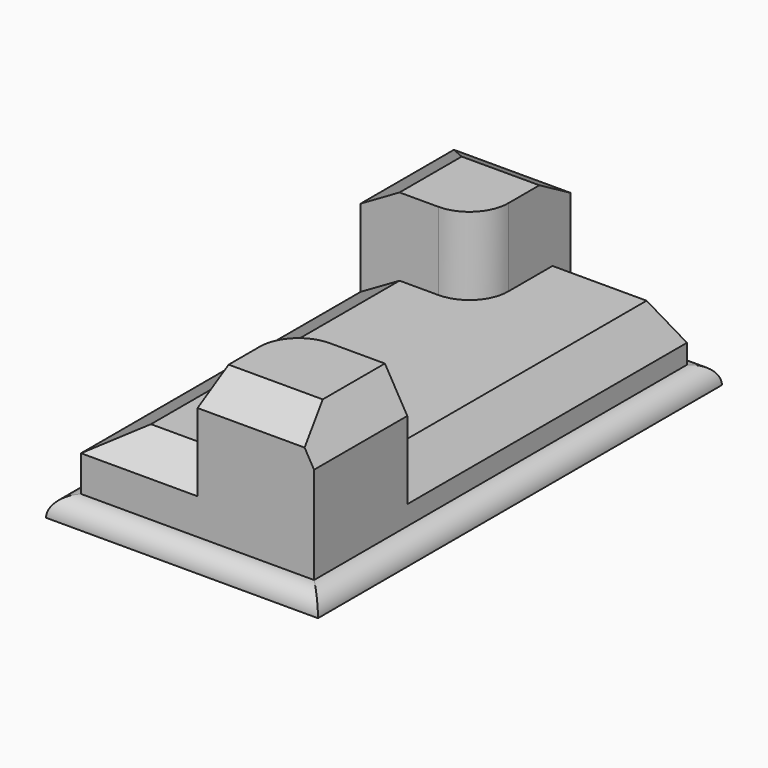
from build123d import *

# Parameters (mm, degrees)
F0_W        = 88.9
F0_H        = 165.1
F1_DEPTH    = 6.35
F2_DEPTH    = 25.4
F3_DEPTH    = 50.8
F4_R        = 6.34999
F5_C1_SIZE2 = 12.7
F5_C1_SIZE  = 7.3323484187
F5_C2_SIZE2 = 12.7
F5_C2_SIZE  = 7.3323484187
F5_C3_SIZE2 = 7.3323484187
F5_C3_SIZE  = 12.7
F5_C4_SIZE2 = 12.7
F5_C4_SIZE  = 7.3323484187
F5_C5_SIZE2 = 7.3323484187
F5_C5_SIZE  = 12.7
F5_C6_SIZE2 = 7.3323484187
F5_C6_SIZE  = 12.7
F5_C7_SIZE2 = 12.7
F5_C7_SIZE  = 7.3323484187
F5_C8_SIZE2 = 12.7
F5_C8_SIZE  = 7.3323484187


# Not quite as in the source:
# - a fillet or chamfer is up to 0.001 mm smaller than in the source, because OpenCascade refuses the exact size


with BuildPart() as f1:
    # F0 (on Top) → F1 (new body)
    with BuildSketch(Plane.XY):
        with Locations((-54.6394883871, -5.459120968)):
            Rectangle(F0_W, F0_H)
        Polygon((-92.7394883871, 32.640879032), (-92.7394883871, 70.740879032), (-54.6394883871, 70.740879032), (-16.5394883871, 70.740879032), (-16.5394883871, -43.559120968), (-16.5394883871, -81.659120968), (-54.6394883871, -81.659120968), (-92.7394883871, -81.659120968), align=None, mode=Mode.SUBTRACT)
    extrude(amount=F1_DEPTH)

    # F0 (on Top) → F2 (join)
    with BuildSketch(Plane.XY):
        with BuildLine():
            Line((-16.5394883871, 70.740879032), (-54.6394883871, 70.740879032))
            Line((-54.6394883871, 70.740879032), (-54.6394883871, 45.340879032))
            ThreePointArc((-54.6394883871, 45.340879032), (-58.359232266, 36.3606229109), (-67.3394883871, 32.640879032))
            Line((-67.3394883871, 32.640879032), (-92.7394883871, 32.640879032))
            Line((-92.7394883871, 32.640879032), (-92.7394883871, -81.659120968))
            Line((-92.7394883871, -81.659120968), (-54.6394883871, -81.659120968))
            Line((-54.6394883871, -81.659120968), (-54.6394883871, -56.259120968))
            ThreePointArc((-54.6394883871, -56.259120968), (-50.9197445082, -47.2788648469), (-41.9394883871, -43.559120968))
            Line((-41.9394883871, -43.559120968), (-16.5394883871, -43.559120968))
            Line((-16.5394883871, -43.559120968), (-16.5394883871, 70.740879032))
        make_face()
    extrude(amount=F2_DEPTH)

    # F0 (on Top) → F3 (join)
    with BuildSketch(Plane.XY):
        with BuildLine():
            Line((-54.6394883871, 70.740879032), (-92.7394883871, 70.740879032))
            Line((-92.7394883871, 70.740879032), (-92.7394883871, 32.640879032))
            Line((-92.7394883871, 32.640879032), (-67.3394883871, 32.640879032))
            ThreePointArc((-67.3394883871, 32.640879032), (-58.359232266, 36.3606229109), (-54.6394883871, 45.340879032))
            Line((-54.6394883871, 45.340879032), (-54.6394883871, 70.740879032))
        make_face()
        with BuildLine():
            Line((-16.5394883871, -81.659120968), (-16.5394883871, -43.559120968))
            Line((-16.5394883871, -43.559120968), (-41.9394883871, -43.559120968))
            ThreePointArc((-41.9394883871, -43.559120968), (-50.9197445082, -47.2788648469), (-54.6394883871, -56.259120968))
            Line((-54.6394883871, -56.259120968), (-54.6394883871, -81.659120968))
            Line((-54.6394883871, -81.659120968), (-16.5394883871, -81.659120968))
        make_face()
    extrude(amount=F3_DEPTH)

    # F4 (radius 6.35 in the source; OpenCascade refuses exactly that, so slightly less here)
    f4_edges = [f1.edges().sort_by_distance(p)[0] for p in [
        (-99.089488, -5.459121, 6.35),
        (-54.639488, -88.009121, 6.35),
        (-10.189488, -5.459121, 6.35),
        (-54.639488, 77.090879, 6.35),
    ]]
    fillet(f4_edges, radius=F4_R)

    # F5: chamfer of 12.7 x 7.3323484187 on 8 edges, made by hand

    # F5_c1
    f5_c1_edges = [f1.edges().sort_by_distance(p)[0] for p in [
        (-92.7394883871, 51.690879032, 50.8),
    ]]
    f5_c1_side = f1.faces().sort_by_distance((-92.7394883871, 51.690879032, 50.6533530316))[0]
    chamfer(f5_c1_edges, length=F5_C1_SIZE, length2=F5_C1_SIZE2, reference=f5_c1_side)

    # F5_c2
    f5_c2_edges = [f1.edges().sort_by_distance(p)[0] for p in [
        (-92.7394883871, -24.509120968, 25.4),
    ]]
    f5_c2_side = f1.faces().sort_by_distance((-92.7394883871, -24.509120968, 25.2533530316))[0]
    chamfer(f5_c2_edges, length=F5_C2_SIZE, length2=F5_C2_SIZE2, reference=f5_c2_side)

    # F5_c3
    f5_c3_edges = [f1.edges().sort_by_distance(p)[0] for p in [
        (-35.5894883871, 70.740879032, 25.4),
    ]]
    f5_c3_side = f1.faces().sort_by_distance((-35.5894883871, 70.740879032, 25.2533530316))[0]
    chamfer(f5_c3_edges, length=F5_C3_SIZE, length2=F5_C3_SIZE2, reference=f5_c3_side)

    # F5_c4
    f5_c4_edges = [f1.edges().sort_by_distance(p)[0] for p in [
        (-67.3394883871, 70.740879032, 50.8),
    ]]
    f5_c4_side = f1.faces().sort_by_distance((-67.3394883871, 70.740879032, 50.6533530316))[0]
    chamfer(f5_c4_edges, length=F5_C4_SIZE, length2=F5_C4_SIZE2, reference=f5_c4_side)

    # F5_c5
    f5_c5_edges = [f1.edges().sort_by_distance(p)[0] for p in [
        (-16.5394883871, -62.609120968, 50.8),
    ]]
    f5_c5_side = f1.faces().sort_by_distance((-16.5394883871, -62.609120968, 50.6533530316))[0]
    chamfer(f5_c5_edges, length=F5_C5_SIZE, length2=F5_C5_SIZE2, reference=f5_c5_side)

    # F5_c6
    f5_c6_edges = [f1.edges().sort_by_distance(p)[0] for p in [
        (-16.5394883871, 9.9247048227, 25.4),
    ]]
    f5_c6_side = f1.faces().sort_by_distance((-16.5394883871, 9.9247048227, 25.2533530316))[0]
    chamfer(f5_c6_edges, length=F5_C6_SIZE, length2=F5_C6_SIZE2, reference=f5_c6_side)

    # F5_c7
    f5_c7_edges = [f1.edges().sort_by_distance(p)[0] for p in [
        (-67.3394883871, -81.659120968, 25.4),
    ]]
    f5_c7_side = f1.faces().sort_by_distance((-67.3394883871, -81.659120968, 25.2533530316))[0]
    chamfer(f5_c7_edges, length=F5_C7_SIZE, length2=F5_C7_SIZE2, reference=f5_c7_side)

    # F5_c8
    f5_c8_edges = [f1.edges().sort_by_distance(p)[0] for p in [
        (-39.2556625965, -81.659120968, 50.8),
    ]]
    f5_c8_side = f1.faces().sort_by_distance((-39.2556625965, -81.659120968, 50.6533530316))[0]
    chamfer(f5_c8_edges, length=F5_C8_SIZE, length2=F5_C8_SIZE2, reference=f5_c8_side)


solid = f1.part
